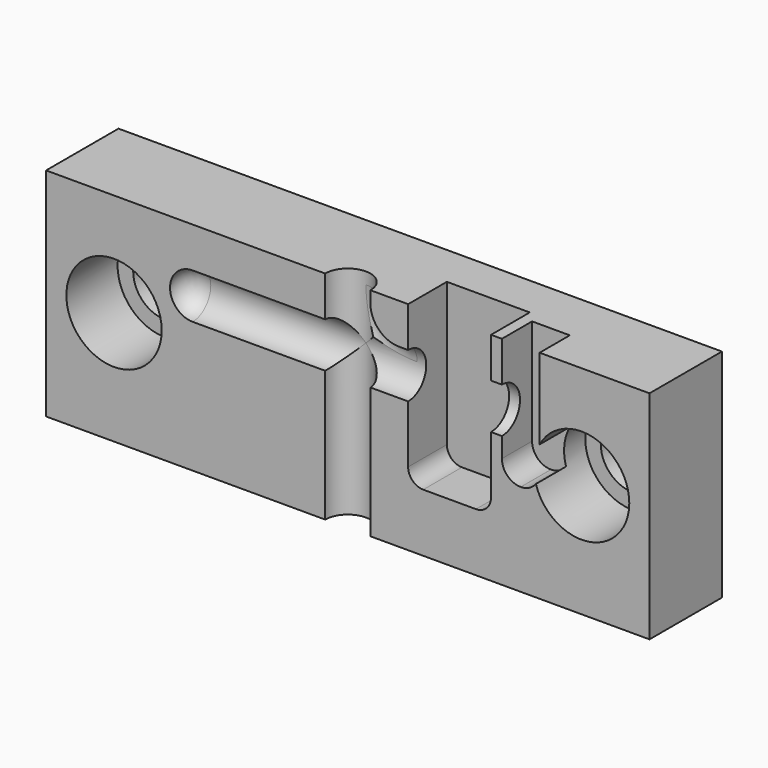
from build123d import *

# Parameters (mm, degrees)
F0_W           = 127
F0_H           = 45.593
F1_DEPTH       = 19.05
F3_D           = 13.5128
F3_DEPTH       = 19.05
F3_CBORE_D     = 20.066
F3_CBORE_DEPTH = 13.4874
F3_TIP         = 4.0596546864
F5_DEPTH       = 45.593
F7_DEPTH       = 10.1854
F9_DEPTH       = 7.9375
F10_R          = 4.7625
F11_DEPTH      = 69.85
F12_R          = 4.76249
F4_R           = 4.7625


# Not quite as in the source:
# - a fillet or chamfer is up to 0.001 mm smaller than in the source, because OpenCascade refuses the exact size


with BuildPart() as f1:
    # F0 (on Front) → F1 (new body)
    with BuildSketch(Plane.XZ):
        with Locations((63.5, -22.7965)):
            Rectangle(F0_W, F0_H)
    extrude(amount=-F1_DEPTH)

    # F3
    with Locations(Plane.XZ):
        with Locations((14.3002, -21.7424), (112.7125, -21.7424)):
            CounterBoreHole(F3_D / 2, F3_CBORE_D / 2, F3_CBORE_DEPTH, depth=F3_DEPTH)
            with Locations((0, 0, -(F3_DEPTH + F3_TIP / 2))):  # 118° drill point
                Cone(0, F3_D / 2, F3_TIP, mode=Mode.SUBTRACT)

    # F4 (on face) → F5 (cut)
    with BuildSketch(Plane.XY):
        with BuildLine():
            Line((58.7375, 0), (68.2625, 0))
            ThreePointArc((68.2625, 0), (63.5, 4.7625), (58.7375, 0))
        make_face()
        with BuildLine():
            ThreePointArc((58.7375, 0), (63.5, -4.7625), (68.2625, 0))
            Line((68.2625, 0), (58.7375, 0))
        make_face()
    extrude(amount=-F5_DEPTH, mode=Mode.SUBTRACT)

    # F6 (on face) → F7 (cut)
    with BuildSketch(Plane.XZ):
        with BuildLine():
            Line((93.6498, 0), (76.2, 0))
            Line((76.2, 0), (76.2, -30.1625))
            ThreePointArc((76.2, -30.1625), (77.1299359697, -32.4075640303), (79.375, -33.3375))
            Line((79.375, -33.3375), (90.4748, -33.3375))
            ThreePointArc((90.4748, -33.3375), (92.7198640303, -32.4075640303), (93.6498, -30.1625))
            Line((93.6498, -30.1625), (93.6498, 0))
        make_face()
    extrude(amount=-F7_DEPTH, mode=Mode.SUBTRACT)

    # F8 (on Front) → F9 (cut)
    with BuildSketch(Plane.XZ):
        with BuildLine():
            Line((103.8733, 0), (95.9358, 0))
            Line((95.9358, 0), (95.9358, -22.1996))
            ThreePointArc((95.9358, -22.1996), (97.0963600902, -25.0014399098), (99.8982, -26.162))
            Line((99.8982, -26.162), (99.9109, -26.162))
            ThreePointArc((99.9109, -26.162), (102.7127399098, -25.0014399098), (103.8733, -22.1996))
            Line((103.8733, -22.1996), (103.8733, 0))
        make_face()
    extrude(amount=-F9_DEPTH, mode=Mode.SUBTRACT)

    # F10 (on face) → F11 (cut)
    with BuildSketch(Plane.YZ.offset(95.9358)):
        with Locations((0, -13.2588)):
            Circle(F10_R)
    extrude(amount=-F11_DEPTH, mode=Mode.SUBTRACT)

    # F12 (radius 4.7625 in the source; OpenCascade refuses exactly that, so slightly less here)
    f12_edges = [f1.edges().sort_by_distance(p)[0] for p in [
        (26.0858, 4.7625, -13.2588),
    ]]
    fillet(f12_edges, radius=F12_R)

    # F14: sweep along a path in F13
    with BuildLine(Plane.XZ) as f14_path:
        Line((63.5, 0), (63.5, -2.4638))
        ThreePointArc((63.5, -2.4638), (66.6617822971, -10.0970177029), (74.295, -13.2588))
        Line((74.295, -13.2588), (77.6987022404, -13.2588))
    # F4 (on face) → F14 (sweep, cut)
    with BuildSketch(Plane.XY):
        with Locations((63.5, 0)):
            Circle(F4_R)
    sweep(path=f14_path.line, mode=Mode.SUBTRACT)


solid = f1.part
